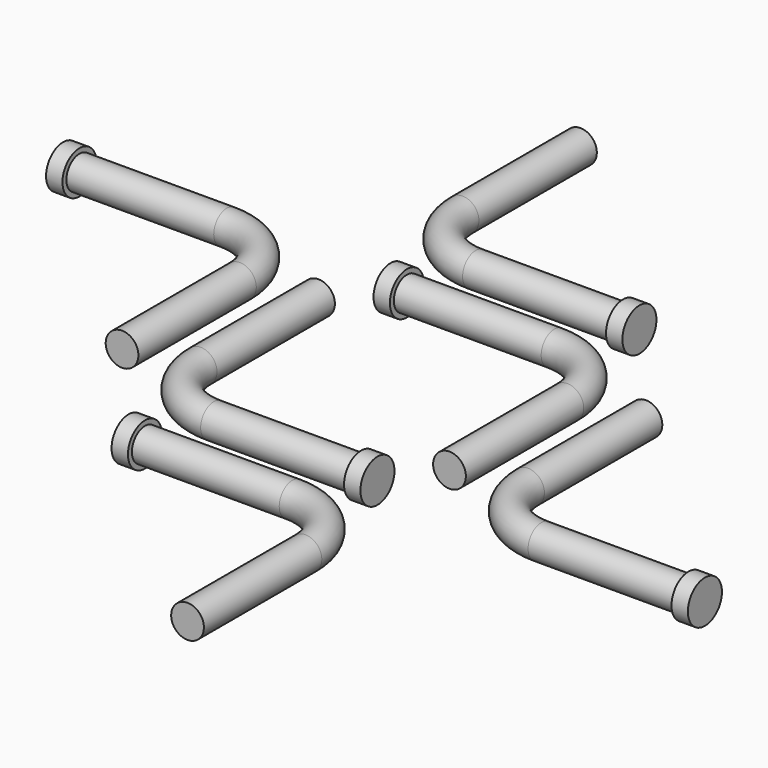
from build123d import *

# Parameters (mm, degrees)
F2_R             = 12.7
F3_COPIES2_COUNT = 2
F9_R             = 12.7
F12_R            = 16.51
F12_R_2          = 12.7
F13_DEPTH        = 12.7
F14_R            = 16.51
F15_DEPTH        = 12.7
F16_R            = 16.51
F17_DEPTH        = 12.7
F18_R            = 16.51
F19_DEPTH        = 12.7
F20_R            = 16.51
F21_DEPTH        = 12.7
F22_R            = 16.51
F22_R_2          = 12.7
F23_DEPTH        = 12.7


# Not quite as in the source:
# - a feature of the source that left no trace in its solid (it failed there, or was rolled back) is left out
# - a pattern or mirror of a feature is missing from the dataset's text; its kind, count and spacing are read off the source's solid


with BuildPart() as f3:
    # F3: sweep along a path in F0
    with BuildLine(Plane.XY) as f3_path:
        Line((-101.6, 317.5), (-101.6, 203.2))
        ThreePointArc((-101.6, 203.2), (-86.7210244843, 167.2789755157), (-50.8, 152.4))
        Line((-50.8, 152.4), (63.5, 152.4))
    # F2 (on plane+point) → F3 (sweep)
    with BuildSketch(Plane.XZ.offset(-317.5)):
        with Locations((-101.6, 0)):
            Circle(F2_R)
    sweep(path=f3_path.line)


with BuildPart() as f3_copies_1:
    # F3_copies: instance of F3
    add(f3.part.mirror(Plane(origin=(0, 0, 0), x_dir=(-0.7071067812, 0.7071067812, 0), z_dir=(-0.7071067812, -0.7071067812, 0))))


with BuildPart() as f3_copies1_1:
    # F3_copies1: instance of F3
    add(f3.part.mirror(Plane(origin=(0, 0, 0), x_dir=(0.7071067812, 0.7071067812, 0), z_dir=(0.7071067812, -0.7071067812, 0))))


with BuildPart() as f3_copies2_1:
    # F3_copies2: instance of F3
    add(f3.part.rotate(Axis((0, 0, 0), (0, 0, 1)), 1 * 360 / F3_COPIES2_COUNT))


with BuildPart() as f10:
    # F10: sweep along a path in F0
    with BuildLine(Plane.XY) as f10_path:
        Line((101.6, -63.5), (101.6, 50.8))
        ThreePointArc((101.6, 50.8), (86.7210244843, 86.7210244843), (50.8, 101.6))
        Line((50.8, 101.6), (-63.5, 101.6))
    # F9 (on plane+point) → F10 (sweep)
    with BuildSketch(Plane.XZ.offset(63.5)):
        with Locations((101.6, 0)):
            Circle(F9_R)
    sweep(path=f10_path.line)


with BuildPart() as f10_copies_1:
    # F10_copies: instance of F10
    add(f10.part.mirror(Plane(origin=(0, 0, 0), x_dir=(-0.7071067812, 0.7071067812, 0), z_dir=(-0.7071067812, -0.7071067812, 0))))


with BuildPart() as f13:
    # F12 (on face) → F13 (new body)
    with BuildSketch(Plane.YZ.offset(63.5)):
        with Locations((152.4, 0)):
            Circle(F12_R)
        with Locations((152.4, 0)):
            Circle(F12_R_2, mode=Mode.SUBTRACT)
        with Locations((152.4, 0)):
            Circle(F12_R_2)
    extrude(amount=F13_DEPTH)


with BuildPart() as f15:
    # F14 (on face) → F15 (new body)
    with BuildSketch(Plane.YZ.offset(317.5)):
        with Locations((-101.6, 0)):
            Circle(F14_R)
    extrude(amount=F15_DEPTH)


with BuildPart() as f17:
    # F16 (on face) → F17 (new body)
    with BuildSketch(Plane.YZ.offset(63.5)):
        with Locations((-101.6, 0)):
            Circle(F16_R)
    extrude(amount=F17_DEPTH)


with BuildPart() as f19:
    # F18 (on face) → F19 (new body)
    with BuildSketch(Plane(origin=(-63.5, 0, 0), x_dir=(0, -1, 0), z_dir=(-1, 0, 0))):
        with Locations((152.4, 0)):
            Circle(F18_R)
    extrude(amount=F19_DEPTH)


with BuildPart() as f21:
    # F20 (on face) → F21 (new body)
    with BuildSketch(Plane(origin=(-317.5, 0, 0), x_dir=(0, -1, 0), z_dir=(-1, 0, 0))):
        with Locations((-101.6, 0)):
            Circle(F20_R)
    extrude(amount=F21_DEPTH)


with BuildPart() as f23:
    # F22 (on face) → F23 (new body)
    with BuildSketch(Plane(origin=(-63.5, 0, 0), x_dir=(0, -1, 0), z_dir=(-1, 0, 0))):
        with Locations((-101.6, 0)):
            Circle(F22_R)
        with Locations((-101.6, 0)):
            Circle(F22_R_2, mode=Mode.SUBTRACT)
        with Locations((-101.6, 0)):
            Circle(F22_R_2)
    extrude(amount=F23_DEPTH)


solid = Compound([f3.part, f3_copies_1.part, f3_copies1_1.part, f3_copies2_1.part, f10.part, f10_copies_1.part, f13.part, f15.part, f17.part, f19.part, f21.part, f23.part])
